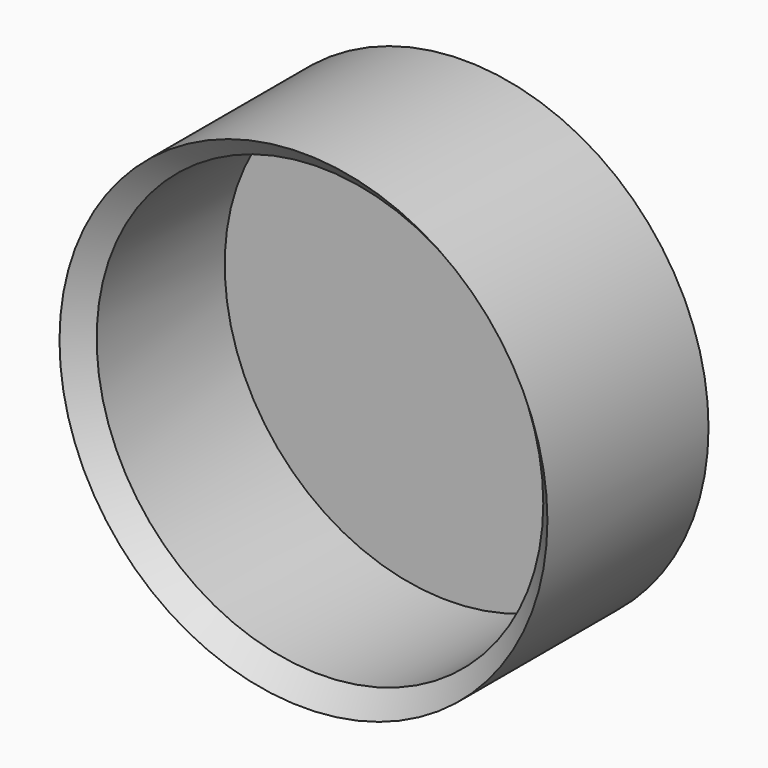
from build123d import *

# Parameters (mm, degrees)
F0_R     = 9.45
F0_R_2   = 8.65
F1_DEPTH = 8
F2_R     = 8.65
F3_DEPTH = 0.8


# Not quite as in the source:
# - a fillet or chamfer that OpenCascade refuses, or shapes differently, is made with other operations: its cross-section is extruded or revolved along the edge and cut away or added


with BuildPart() as f1:
    # F0 (on Front) → F1 (new body)
    with BuildSketch(Plane.XZ):
        Circle(F0_R)
        Circle(F0_R_2, mode=Mode.SUBTRACT)
    extrude(amount=F1_DEPTH)

    # F2 (on Front) → F3 (join)
    with BuildSketch(Plane.XZ):
        Circle(F2_R)
    extrude(amount=F3_DEPTH)

    # F4: chamfer of 1 on 1 edges, made by hand

    # F4_s1 → F4_t2 (revolve, cut)
    with BuildSketch(Plane.XY):
        Polygon((9.65, -8), (8.65, -7), (8.65, -8), align=None)
    revolve(axis=Axis((0, -8, 0), (0, -1, 0)), mode=Mode.SUBTRACT)


solid = f1.part
